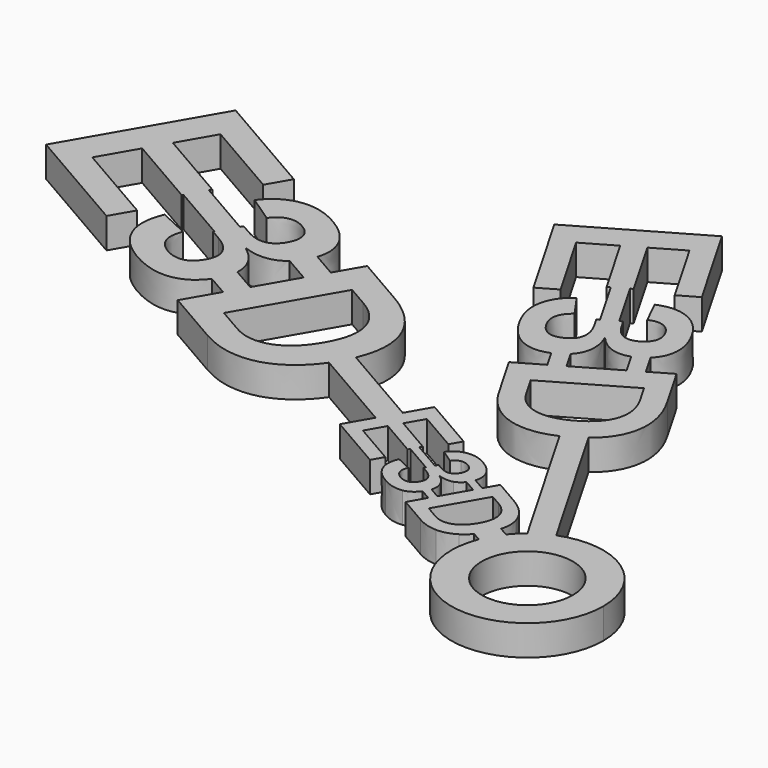
from build123d import *

# Parameters (mm, degrees)
F0_TEXT_SIZE   = 15.2079207921
F0_R           = 3
F0_TEXT_SIZE_2 = 12.6732673267
F1_DEPTH       = 2


# Not quite as in the source:
# - Text() gives the source's letters only with a copy of the font that has no kerning and outlines rounded to 1/6400 em; it was checked with that copy


with BuildPart() as f1:
    # F0 (on Top) → F1 (new body)
    with BuildSketch(Plane.XY):
        with BuildLine():
            Line((-29.1540964549, 20.2671880477), (-30.7902893261, 21.2118444423))
            add(Edge.make_bspline(
                [(-30.7902893261, 21.2118444423), (-30.8857444527, 20.9320441506), (-31.0483473531, 20.6504076656)],
                knots=[0.7511682888, 0.7511682888, 0.7511682888, 1, 1, 1], degree=2))
            add(Edge.make_bspline(
                [(-31.0483473531, 20.6504076656), (-31.2909550672, 20.2301987785), (-31.6127128534, 19.9546200797)],
                knots=[0, 0, 0, 0.494418465, 0.494418465, 0.494418465], degree=2))
            Line((-31.6127128534, 19.9546200797), (-29.9040964549, 18.9681499421))
            Line((-29.9040964549, 18.9681499421), (-29.1540964549, 20.2671880477))
        make_face()
        with BuildLine():
            Line((-32.1289479401, 15.1145941305), (-31.3789479401, 16.4136322362))
            Line((-31.3789479401, 16.4136322362), (-32.9437034814, 17.3170442691))
            add(Edge.make_bspline(
                [(-32.9437034814, 17.3170442691), (-32.975793504, 16.7796957758), (-33.2832110872, 16.2472329024)],
                knots=[0.3911926292, 0.3911926292, 0.3911926292, 1, 1, 1], degree=2))
            add(Edge.make_bspline(
                [(-33.2832110872, 16.2472329024), (-33.3875153345, 16.0665726466), (-33.5018976995, 15.9072670437)],
                knots=[0, 0, 0, 0.1418245689, 0.1418245689, 0.1418245689], degree=2))
            Line((-33.5018976995, 15.9072670437), (-32.1289479401, 15.1145941305))
        make_face()
        with BuildLine():
            Line((-16.5114084248, 10.3843720007), (-22.2409058517, 13.6922988825))
            add(Edge.make_bspline(
                [(-22.2409058517, 13.6922988825), (-22.4111389258, 13.292867735), (-22.647503085, 12.8834730021)],
                knots=[0.8099906075, 0.8099906075, 0.8099906075, 1, 1, 1], degree=2))
            add(Edge.make_bspline(
                [(-22.647503085, 12.8834730021), (-22.8002351075, 12.6189333792), (-22.965200333, 12.3784196886)],
                knots=[0, 0, 0, 0.1887657156, 0.1887657156, 0.1887657156], degree=2))
            Line((-22.965200333, 12.3784196886), (-17.2614084248, 9.0853338951))
            Line((-17.2614084248, 9.0853338951), (-16.5114084248, 10.3843720007))
        make_face()
        Polygon((-15.633190603, 11.9054898882), (-16.5114084248, 10.3843720007), (-16.1779665272, 10.1918592314), (-16.9279665272, 8.8928211257), (-17.2614084248, 9.0853338951), (-18.2488341674, 7.3750623402), (-14.5539067714, 5.2417950135), (-14.1303424149, 5.9754299991), (-16.8765861409, 7.5609745536), (-16.1880712894, 8.7535172581), (-13.770059766, 7.3574776541), (-13.6947132313, 7.4879816803), (-13.4447132313, 7.9209943822), (-13.347089469, 8.0900836987), (-15.7651009924, 9.4861233026), (-15.10747723, 10.6251610713), (-12.4929379615, 9.1156561209), (-12.0699676645, 9.8482621654), align=None)
        Polygon((-16.1779665272, 10.1918592314), (-16.5114084248, 10.3843720007), (-17.2614084248, 9.0853338951), (-16.9279665272, 8.8928211257), align=None)
        Polygon((-11.544259068, 6.8237666595), (-13.4447132313, 7.9209943822), (-13.6947132313, 7.4879816803), (-11.794259068, 6.3907539576), align=None)
        Polygon((-36.6829324931, 20.1013169534), (-35.9788991928, 21.3207383997), (-39.7798075194, 23.5151938452), (-40.4838408197, 22.2957723989), align=None)
        with BuildLine():
            Line((-11.4424768898, 7.0000585634), (-11.544259068, 6.8237666595))
            Line((-11.544259068, 6.8237666595), (-11.794259068, 6.3907539576))
            Line((-11.794259068, 6.3907539576), (-11.864259068, 6.269510401))
            Line((-11.864259068, 6.269510401), (-11.5494030994, 6.0877282228))
            add(Edge.make_bspline(
                [(-10.9923000787, 5.5520649004), (-11.1182767895, 5.8388173317), (-11.5494030994, 6.0877282228)],
                knots=[0, 0, 0, 1, 1, 1], degree=2))
            add(Edge.make_bspline(
                [(-11.0409768331, 4.9628037935), (-10.8663233678, 5.2653124692), (-10.9923000787, 5.5520649004)],
                knots=[0, 0, 0, 1, 1, 1], degree=2))
            add(Edge.make_bspline(
                [(-11.5050019171, 4.5749303562), (-11.2322639619, 4.6314847677), (-11.0409768331, 4.9628037935)],
                knots=[0, 0, 0, 1, 1, 1], degree=2))
            add(Edge.make_bspline(
                [(-12.1018563106, 4.7055046576), (-11.7777398723, 4.5183759448), (-11.5050019171, 4.5749303562)],
                knots=[0, 0, 0, 1, 1, 1], degree=2))
            add(Edge.make_bspline(
                [(-12.4681181025, 5.7867641895), (-12.7583207157, 5.0845145586), (-12.1018563106, 4.7055046576)],
                knots=[0, 0, 0, 1, 1, 1], degree=2))
            Line((-12.4681181025, 5.7867641895), (-13.4343280561, 6.2375958947))
            add(Edge.make_bspline(
                [(-13.4895334495, 4.976432794), (-13.7261848929, 5.560995916), (-13.4343280561, 6.2375958947)],
                knots=[0, 0, 0, 1, 1, 1], degree=2))
            add(Edge.make_bspline(
                [(-12.5223338438, 3.9700874938), (-13.2528820062, 4.391869672), (-13.4895334495, 4.976432794)],
                knots=[0, 0, 0, 1, 1, 1], degree=2))
            add(Edge.make_bspline(
                [(-11.132382913, 3.6306224329), (-11.7506280384, 3.5245429393), (-12.5223338438, 3.9700874938)],
                knots=[0, 0, 0, 1, 1, 1], degree=2))
            add(Edge.make_bspline(
                [(-10.2557583214, 4.2036335218), (-10.6018201359, 3.7216572481), (-11.132382913, 3.6306224329)],
                knots=[0.1418245689, 0.1418245689, 0.1418245689, 1, 1, 1], degree=2))
            add(Edge.make_bspline(
                [(-10.1464150152, 4.3736164512), (-10.1985671389, 4.2832863233), (-10.2557583214, 4.2036335218)],
                knots=[0, 0, 0, 0.1418245689, 0.1418245689, 0.1418245689], degree=2))
            add(Edge.make_bspline(
                [(-10.0248577478, 4.6476732827), (-10.0674875561, 4.5103228205), (-10.1464150152, 4.3736164512)],
                knots=[0.687385358, 0.687385358, 0.687385358, 1, 1, 1], degree=2))
            add(Edge.make_bspline(
                [(-10.0128799039, 5.2548070388), (-9.9311221958, 4.9496831183), (-10.0248577478, 4.6476732827)],
                knots=[0, 0, 0, 0.687385358, 0.687385358, 0.687385358], degree=2))
            add(Edge.make_bspline(
                [(-10.6174147184, 6.0599992528), (-10.13182004, 5.69869767), (-10.0128799039, 5.2548070388)],
                knots=[0, 0, 0, 1, 1, 1], degree=2))
            Line((-10.6174147184, 6.0599992528), (-10.6096919461, 6.0733754867))
            add(Edge.make_bspline(
                [(-9.6815706655, 6.0211267202), (-10.0888116482, 5.892002271), (-10.6096919461, 6.0733754867)],
                knots=[0, 0, 0, 1, 1, 1], degree=2))
            add(Edge.make_bspline(
                [(-9.1354956255, 6.4145618951), (-9.3571681192, 6.1239854743), (-9.6815706655, 6.0211267202)],
                knots=[0.2034138014, 0.2034138014, 0.2034138014, 1, 1, 1], degree=2))
            add(Edge.make_bspline(
                [(-9.0289831482, 6.5752038328), (-9.0788900194, 6.4887625961), (-9.1354956255, 6.4145618951)],
                knots=[0, 0, 0, 0.2034138014, 0.2034138014, 0.2034138014], degree=2))
            add(Edge.make_bspline(
                [(-8.8999541346, 6.8559222212), (-8.947681698, 6.7160220753), (-9.0289831482, 6.5752038328)],
                knots=[0.7511682888, 0.7511682888, 0.7511682888, 1, 1, 1], degree=2))
            add(Edge.make_bspline(
                [(-8.9177560774, 7.6922112063), (-8.7558751027, 7.2782500371), (-8.8999541346, 6.8559222212)],
                knots=[0, 0, 0, 0.7511682888, 0.7511682888, 0.7511682888], degree=2))
            add(Edge.make_bspline(
                [(-9.8442599618, 8.6537960386), (-9.1332616798, 8.2433009891), (-8.9177560774, 7.6922112063)],
                knots=[0, 0, 0, 1, 1, 1], degree=2))
            add(Edge.make_bspline(
                [(-11.1190220413, 8.9480215673), (-10.5130716598, 9.0399346525), (-9.8442599618, 8.6537960386)],
                knots=[0, 0, 0, 1, 1, 1], degree=2))
            add(Edge.make_bspline(
                [(-12.1339891588, 8.3116311102), (-11.7249724227, 8.8561084822), (-11.1190220413, 8.9480215673)],
                knots=[0, 0, 0, 1, 1, 1], degree=2))
            Line((-12.1339891588, 8.3116311102), (-11.2674105792, 7.7262526052))
            add(Edge.make_bspline(
                [(-10.8173786455, 8.0494931556), (-11.0783207157, 7.9943599153), (-11.2674105792, 7.7262526052)],
                knots=[0, 0, 0, 1, 1, 1], degree=2))
            add(Edge.make_bspline(
                [(-10.2765646032, 7.9430422375), (-10.5564365752, 8.1046263959), (-10.8173786455, 8.0494931556)],
                knots=[0, 0, 0, 1, 1, 1], degree=2))
            add(Edge.make_bspline(
                [(-9.9133373859, 7.5206850839), (-9.9771427507, 7.7701709503), (-10.2765646032, 7.9430422375)],
                knots=[0, 0, 0, 1, 1, 1], degree=2))
            add(Edge.make_bspline(
                [(-10.0105221202, 6.9923561865), (-9.8495320212, 7.2711992175), (-9.9133373859, 7.5206850839)],
                knots=[0, 0, 0, 1, 1, 1], degree=2))
            add(Edge.make_bspline(
                [(-10.4694066819, 6.6502180781), (-10.1816112291, 6.6960211572), (-10.0105221202, 6.9923561865)],
                knots=[0, 0, 0, 1, 1, 1], degree=2))
            add(Edge.make_bspline(
                [(-11.1461418605, 6.8289694545), (-10.7572021346, 6.6044149991), (-10.4694066819, 6.6502180781)],
                knots=[0, 0, 0, 1, 1, 1], degree=2))
            Line((-11.1461418605, 6.8289694545), (-11.4424768898, 7.0000585634))
        make_face()
        with Locations(Location((-50.3688229507, 22.7586395319), (0, 0, -30))):
            Text('E3D', F0_TEXT_SIZE, font='Arimo', font_style=FontStyle.BOLD, text_align=(TextAlign.LEFT, TextAlign.BOTTOM))
        with BuildLine():
            add(Edge.make_bspline(
                [(-10.1464150152, 4.3736164512), (-10.1985671389, 4.2832863233), (-10.2557583214, 4.2036335218)],
                knots=[0, 0, 0, 0.1418245689, 0.1418245689, 0.1418245689], degree=2))
            Line((-10.2557583214, 4.2036335218), (-9.5692834417, 3.8072970652))
            Line((-9.5692834417, 3.8072970652), (-9.3192834417, 4.2403097671))
            Line((-9.3192834417, 4.2403097671), (-10.0248577478, 4.6476732827))
            add(Edge.make_bspline(
                [(-10.0248577478, 4.6476732827), (-10.0674875561, 4.5103228205), (-10.1464150152, 4.3736164512)],
                knots=[0.687385358, 0.687385358, 0.687385358, 1, 1, 1], degree=2))
        make_face()
        with BuildLine():
            Line((-8.0818576991, 6.3835940239), (-8.8999541346, 6.8559222212))
            add(Edge.make_bspline(
                [(-8.8999541346, 6.8559222212), (-8.947681698, 6.7160220753), (-9.0289831482, 6.5752038328)],
                knots=[0.7511682888, 0.7511682888, 0.7511682888, 1, 1, 1], degree=2))
            add(Edge.make_bspline(
                [(-9.0289831482, 6.5752038328), (-9.0788900194, 6.4887625961), (-9.1354956255, 6.4145618951)],
                knots=[0, 0, 0, 0.2034138014, 0.2034138014, 0.2034138014], degree=2))
            Line((-9.1354956255, 6.4145618951), (-8.3318576991, 5.950581322))
            Line((-8.3318576991, 5.950581322), (-8.0818576991, 6.3835940239))
        make_face()
        with BuildLine():
            Line((-9.3192834417, 4.2403097671), (-9.5692834417, 3.8072970652))
            Line((-9.5692834417, 3.8072970652), (-10.1942834417, 2.7247653105))
            Line((-10.1942834417, 2.7247653105), (-8.3617393892, 1.6667455085))
            add(Edge.make_bspline(
                [(-7.0484944653, 1.2775900633), (-7.7114486306, 1.291299964), (-8.3617393892, 1.6667455085)],
                knots=[0, 0, 0, 1, 1, 1], degree=2))
            add(Edge.make_bspline(
                [(-5.8093278848, 1.6274538962), (-6.3855403, 1.2638801627), (-7.0484944653, 1.2775900633)],
                knots=[0, 0, 0, 1, 1, 1], degree=2))
            add(Edge.make_bspline(
                [(-5.2142805236, 2.1444408601), (-5.4845342999, 1.8323894602), (-5.8093278848, 1.6274538962)],
                knots=[0.4363301167, 0.4363301167, 0.4363301167, 1, 1, 1], degree=2))
            add(Edge.make_bspline(
                [(-4.8285610141, 2.6917365011), (-5.0050803069, 2.3859961175), (-5.2142805236, 2.1444408601)],
                knots=[0, 0, 0, 0.4363301167, 0.4363301167, 0.4363301167], degree=2))
            add(Edge.make_bspline(
                [(-4.4959723962, 3.461776277), (-4.6009346477, 3.0859969328), (-4.8285610141, 2.6917365011)],
                knots=[0.6340295606, 0.6340295606, 0.6340295606, 1, 1, 1], degree=2))
            add(Edge.make_bspline(
                [(-4.5004530738, 4.7083529557), (-4.3141293754, 4.1127993837), (-4.4959723962, 3.461776277)],
                knots=[0, 0, 0, 0.6340295606, 0.6340295606, 0.6340295606], degree=2))
            add(Edge.make_bspline(
                [(-5.9385078057, 6.3082621654), (-4.7943253316, 5.647668106), (-4.5004530738, 4.7083529557)],
                knots=[0, 0, 0, 1, 1, 1], degree=2))
            Line((-5.9385078057, 6.3082621654), (-7.5786398773, 7.2551928585))
            Line((-7.5786398773, 7.2551928585), (-8.0818576991, 6.3835940239))
            Line((-8.0818576991, 6.3835940239), (-8.3318576991, 5.950581322))
            Line((-8.3318576991, 5.950581322), (-9.3192834417, 4.2403097671))
        make_face()
        with BuildLine():
            add(Edge.make_bspline(
                [(-5.7834183306, 3.2430236298), (-5.3616361524, 3.9735717922), (-5.51891975, 4.5767921743)],
                knots=[0, 0, 0, 1, 1, 1], degree=2))
            add(Edge.make_bspline(
                [(-6.8041417658, 2.3067619478), (-6.201042093, 2.5196780549), (-5.7834183306, 3.2430236298)],
                knots=[0, 0, 0, 1, 1, 1], degree=2))
            add(Edge.make_bspline(
                [(-8.0184324365, 2.4467171278), (-7.4072414387, 2.0938458407), (-6.8041417658, 2.3067619478)],
                knots=[0, 0, 0, 1, 1, 1], degree=2))
            Line((-8.0184324365, 2.4467171278), (-8.8220354152, 2.9106775239))
            Line((-8.8220354152, 2.9106775239), (-7.0529265043, 5.9748640416))
            Line((-7.0529265043, 5.9748640416), (-6.3810279831, 5.5869432496))
            add(Edge.make_bspline(
                [(-5.51891975, 4.5767921743), (-5.6762033475, 5.1800125565), (-6.3810279831, 5.5869432496)],
                knots=[0, 0, 0, 1, 1, 1], degree=2))
        make_face(mode=Mode.SUBTRACT)
        with BuildLine():
            Line((-3.9061359474, 3.1212340445), (-4.4959723962, 3.461776277))
            add(Edge.make_bspline(
                [(-4.4959723962, 3.461776277), (-4.6009346477, 3.0859969328), (-4.8285610141, 2.6917365011)],
                knots=[0.6340295606, 0.6340295606, 0.6340295606, 1, 1, 1], degree=2))
            add(Edge.make_bspline(
                [(-4.8285610141, 2.6917365011), (-5.0050803069, 2.3859961175), (-5.2142805236, 2.1444408601)],
                knots=[0, 0, 0, 0.4363301167, 0.4363301167, 0.4363301167], degree=2))
            Line((-5.2142805236, 2.1444408601), (-4.6561359474, 1.8221959388))
            ThreePointArc((-4.6561359474, 1.8221959388), (-4.3301270189, 2.5), (-3.9061359474, 3.1212340445))
        make_face()
        with BuildLine():
            ThreePointArc((-3.1212340445, 3.9061359474), (-3.5355339059, 3.5355339059), (-3.9061359474, 3.1212340445))
            ThreePointArc((-3.9061359474, 3.1212340445), (-4.3301270189, 2.5), (-4.6561359474, 1.8221959388))
            ThreePointArc((-4.6561359474, 1.8221959388), (-0.9271785866, -4.9132819854), (5, 0))
            ThreePointArc((5, 0), (2.8186007438, 4.1298292758), (-1.8221959388, 4.6561359474))
            ThreePointArc((-1.8221959388, 4.6561359474), (-2.5, 4.3301270189), (-3.1212340445, 3.9061359474))
        make_face()
        Circle(F0_R, mode=Mode.SUBTRACT)
        with BuildLine():
            Line((-8.6035539258, 13.4017925251), (-3.1212340445, 3.9061359474))
            ThreePointArc((-3.1212340445, 3.9061359474), (-2.5, 4.3301270189), (-1.8221959388, 4.6561359474))
            Line((-1.8221959388, 4.6561359474), (-7.3209553936, 14.1802667017))
            add(Edge.make_bspline(
                [(-7.3209553936, 14.1802667017), (-7.6535484776, 13.9169516614), (-8.0596470857, 13.6824905207)],
                knots=[0.7738244966, 0.7738244966, 0.7738244966, 1, 1, 1], degree=2))
            add(Edge.make_bspline(
                [(-8.0596470857, 13.6824905207), (-8.332506108, 13.5249552907), (-8.6035539258, 13.4017925251)],
                knots=[0, 0, 0, 0.2336425585, 0.2336425585, 0.2336425585], degree=2))
        make_face()
        with BuildLine():
            Line((-10.4726850622, 21.2639750947), (-9.6066596584, 21.7639750947))
            Line((-9.6066596584, 21.7639750947), (-10.4029070224, 23.1431159845))
            add(Edge.make_bspline(
                [(-10.4029070224, 23.1431159845), (-10.6106232969, 22.9472554575), (-10.8862114337, 22.7881445725)],
                knots=[0.7078145567, 0.7078145567, 0.7078145567, 1, 1, 1], degree=2))
            add(Edge.make_bspline(
                [(-10.8862114337, 22.7881445725), (-11.0696119627, 22.6822582277), (-11.2521509188, 22.614049561)],
                knots=[0, 0, 0, 0.2589472354, 0.2589472354, 0.2589472354], degree=2))
            Line((-11.2521509188, 22.614049561), (-10.4726850622, 21.2639750947))
        make_face()
        with BuildLine():
            Line((-14.7101069932, 20.3539002217), (-14.0448254901, 19.201598857))
            Line((-14.0448254901, 19.201598857), (-13.1788000863, 19.701598857))
            Line((-13.1788000863, 19.701598857), (-13.8681408045, 20.8955720047))
            add(Edge.make_bspline(
                [(-13.8681408045, 20.8955720047), (-14.0648234194, 20.6968800863), (-14.3337415582, 20.5416201265)],
                knots=[0.631029272, 0.631029272, 0.631029272, 1, 1, 1], degree=2))
            add(Edge.make_bspline(
                [(-14.3337415582, 20.5416201265), (-14.5232107729, 20.4322300244), (-14.7101069932, 20.3539002217)],
                knots=[0, 0, 0, 0.1784878888, 0.1784878888, 0.1784878888], degree=2))
        make_face()
        Polygon((-16.8888320396, 27.9770676484), (-15.0601191684, 24.8096440429), (-14.1940937646, 25.3096440429), (-16.0228066359, 28.4770676484), align=None)
        with Locations(Location((-23.9511337234, 32.3598280326), (0, 0, -60))):
            Text('E3D', F0_TEXT_SIZE_2, font='Arimo', font_style=FontStyle.BOLD, text_align=(TextAlign.LEFT, TextAlign.BOTTOM))
    extrude(amount=F1_DEPTH)


solid = f1.part
